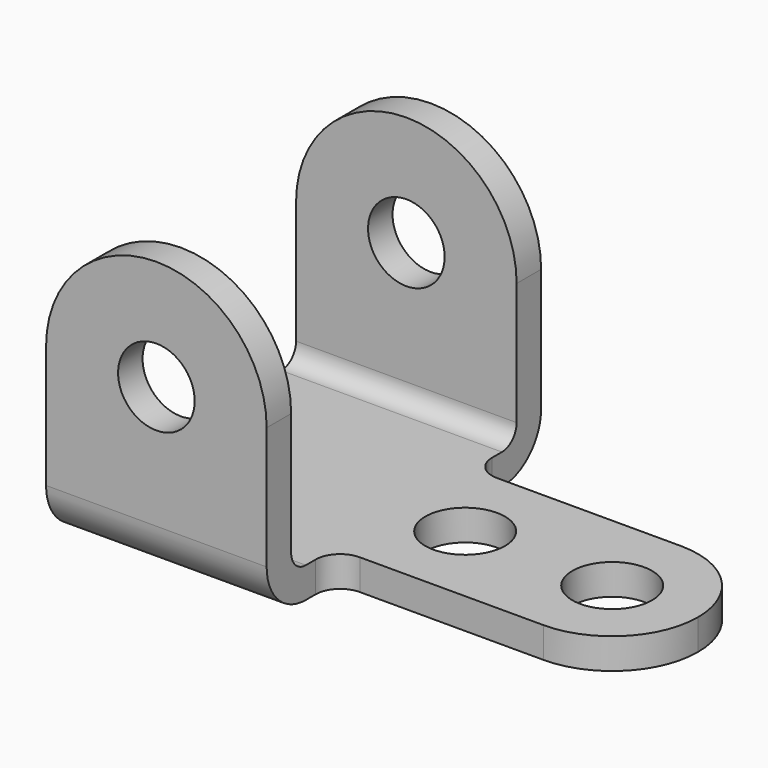
from build123d import *

# Parameters (mm, degrees)
F0_R     = 9.92251
F0_W     = 76.2
F0_H     = 7.9375
F1_DEPTH = 44.45
F2_T     = 7.9375
F3_R     = 10.3251
F4_DEPTH = 7.9385
F5_R     = 6.35
F6_R     = 4.7625
F7_R     = 12.7


# Not quite as in the source:
# - a shell that OpenCascade refuses in one call is made with other operations: the cavity is built on its own and cut out


with BuildPart() as f1:
    # F0 (on Front) → F1 (new body, symmetric)
    with BuildSketch(Plane.XZ):
        with BuildLine():
            ThreePointArc((28.575, 0), (0, 28.575), (-28.575, 0))
            Line((-28.575, 0), (-28.575, -44.45))
            Line((-28.575, -44.45), (28.575, -44.45))
            Line((28.575, -44.45), (28.575, -36.5125))
            Line((28.575, -36.5125), (28.575, 0))
        make_face()
        Circle(F0_R, mode=Mode.SUBTRACT)
        with Locations((66.675, -40.48125)):
            Rectangle(F0_W, F0_H)
    extrude(amount=F1_DEPTH, both=True)

    # F2: shell of thickness 7.9375, made by hand


with BuildPart() as f2_core1:
    # F2_t2: copy of F1
    add(f1.part)

    # the walls: a layer under each face that stays
    f2_faces = [f2_core1.faces().sort_by_distance(p)[0] for p in [
        (66.675, 0, -36.5125),
        (104.775, 0, -40.48125),
        (38.1, 0, -44.45),
        (-6.35, -44.45, -32.2791666667),
        (-6.35, 44.45, -32.2791666667),
    ]]
    thicken(f2_faces, amount=-F2_T, mode=Mode.SUBTRACT)


with BuildPart() as f1_1:
    add(f1.part)

    # what is left inside the walls is the cavity
    f2_cavity = [f2_core1.part.solids().sort_by_distance(p)[0] for p in [
        (0, 12.170833, 28.495625),
    ]]
    add(f2_cavity, mode=Mode.SUBTRACT)

    # F3 (on face) → F4 (cut, through all)
    with BuildSketch(Plane.XY.offset(-36.5125)):
        with Locations((44.45, 0)):
            Circle(F3_R)
        with Locations((82.55, 0)):
            Circle(F3_R)
        with BuildLine():
            Line((104.775, -44.45), (104.775, -6.98e-08))
            ThreePointArc((104.775, -6.98e-08), (98.2654481872, -15.7154482366), (82.55, -22.225))
            Line((82.55, -22.225), (28.575, -22.225))
            Line((28.575, -22.225), (28.575, -44.45))
            Line((28.575, -44.45), (104.775, -44.45))
        make_face()
        with BuildLine():
            Line((28.575, 22.225), (82.55, 22.225))
            ThreePointArc((82.55, 22.225), (98.2654482366, 15.7154481872), (104.775, -6.98e-08))
            Line((104.775, -6.98e-08), (104.775, 44.45))
            Line((104.775, 44.45), (28.575, 44.45))
            Line((28.575, 44.45), (28.575, 22.225))
        make_face()
    extrude(amount=-F4_DEPTH, mode=Mode.SUBTRACT)

    # F5
    f5_edges = [f1_1.edges().sort_by_distance(p)[0] for p in [
        (28.575, -22.225, -40.48125),
        (28.575, 22.225, -40.48125),
    ]]
    fillet(f5_edges, radius=F5_R)

    # F6
    f6_edges = [f1_1.edges().sort_by_distance(p)[0] for p in [
        (0, -36.5125, -36.5125),
        (0, 36.5125, -36.5125),
    ]]
    fillet(f6_edges, radius=F6_R)

    # F7
    f7_edges = [f1_1.edges().sort_by_distance(p)[0] for p in [
        (0, -44.45, -44.45),
        (0, 44.45, -44.45),
    ]]
    fillet(f7_edges, radius=F7_R)


solid = f1_1.part
